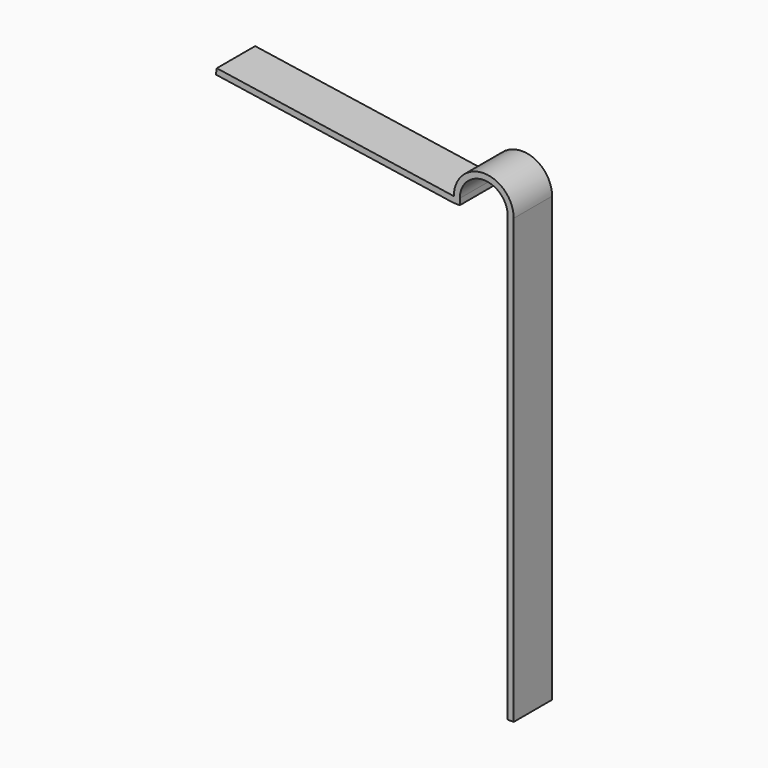
from build123d import *

# Parameters (mm, degrees)
F1_DEPTH = 40


# Not quite as in the source:
# - ends of sketch curves that miss each other by under 0.0002 mm in the source are joined


with BuildPart() as f1:
    # F0 (on Front) → F1 (new body)
    with BuildSketch(Plane.XZ):
        with BuildLine():
            Line((-4.9999998882, 0), (0, 0))
            Line((0, 0), (0, 370))
            ThreePointArc((0, 370), (-25, 395), (-50, 370))
            Line((-50, 370), (-247.7872705737, 399.6680905861))
            Line((-247.7872705737, 399.6680905861), (-248.5289721923, 394.7234131282))
            Line((-248.5289721923, 394.7234131282), (-50, 364.9440672994))
            Line((-50, 364.9440672994), (-45, 364.9440672994))
            Line((-45, 364.9440672994), (-45, 370))
            ThreePointArc((-45, 370), (-25, 390), (-5, 370))
            Line((-5, 370), (-4.9999998882, 0))
        make_face()
    extrude(amount=-F1_DEPTH)


solid = f1.part
